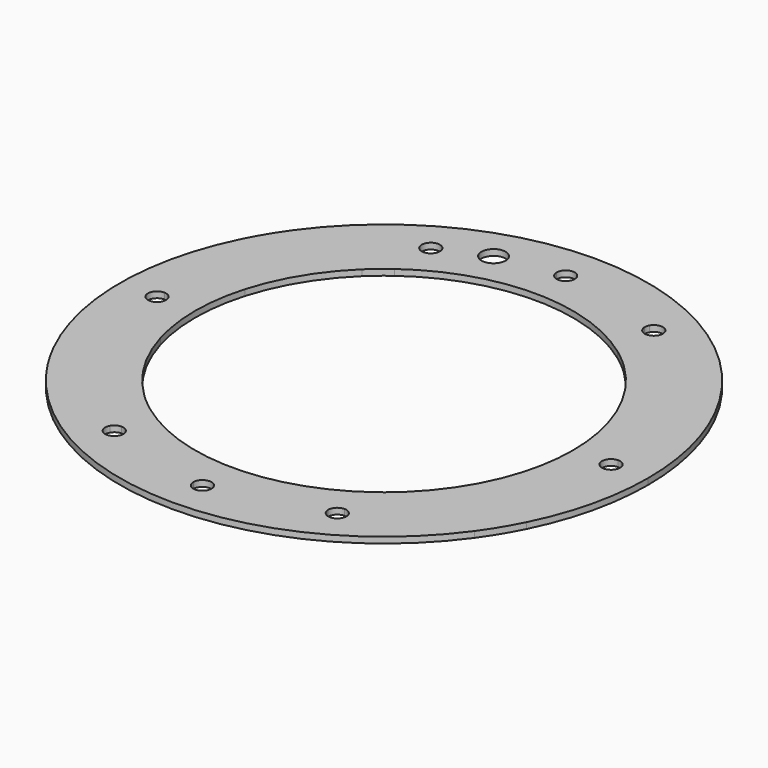
from build123d import *

# Parameters (mm, degrees)
F0_W     = 2.1041625413
F0_H     = 6.15
F1_DEPTH = 2


# Not quite as in the source:
# - a feature names something its author has since deleted; it is built from what else it names


with BuildPart() as f1:
    # F0 (on Top) → F1 (new body)
    with BuildSketch(Plane.XY):
        with Locations((59.2149618303, 40.7632449339)):
            Rectangle(F0_W, F0_H)
        with BuildLine():
            Line((58.1628805597, 43.8382449339), (60.2670431009, 43.8382449339))
            Line((60.2670431009, 43.8382449339), (60.2670431009, 37.6882449339))
            Line((60.2670431009, 37.6882449339), (62.3712056422, 37.6882449339))
            Line((62.3712056422, 37.6882449339), (62.3712056422, 41.1268579364))
            ThreePointArc((62.3712056422, 41.1268579364), (60.3323424952, 43.9759631228), (58.1628805597, 46.7269262644))
            Line((58.1628805597, 46.7269262644), (58.1628805597, 43.8382449339))
        make_face()
        with BuildLine():
            Line((58.1628805597, 37.6882449339), (58.1628805597, 43.8382449339))
            Line((58.1628805597, 43.8382449339), (53.7670431009, 43.8382449339))
            ThreePointArc((53.7670431009, 43.8382449339), (54.9789878574, 40.0585000032), (58.1628805597, 37.6882449339))
        make_face()
        with BuildLine():
            Line((53.7670431009, 43.8382449339), (58.1628805597, 43.8382449339))
            Line((58.1628805597, 43.8382449339), (58.1628805597, 46.7269262644))
            ThreePointArc((58.1628805597, 46.7269262644), (57.217639487, 47.8472580426), (56.25072261, 48.9489366399))
            ThreePointArc((56.25072261, 48.9489366399), (54.4208441995, 46.6793641507), (53.7670431009, 43.8382449339))
        make_face()
        with BuildLine():
            Line((62.3712056422, 37.6882449339), (60.2670431009, 37.6882449339))
            Line((60.2670431009, 37.6882449339), (60.2670431009, 37.3382449339))
            ThreePointArc((60.2670431009, 37.3382449339), (61.3335795513, 37.4263419402), (62.3712056422, 37.6882449339))
        make_face()
        with BuildLine():
            Line((60.2670431009, 37.3382449339), (60.2670431009, 37.6882449339))
            Line((60.2670431009, 37.6882449339), (58.1628805597, 37.6882449339))
            ThreePointArc((58.1628805597, 37.6882449339), (59.2005066506, 37.4263419402), (60.2670431009, 37.3382449339))
        make_face()
        with BuildLine():
            ThreePointArc((58.1628805597, 37.6882449339), (54.9789878574, 40.0585000032), (53.7670431009, 43.8382449339))
            Line((53.7670431009, 43.8382449339), (43.6404220332, 43.8382449339))
            ThreePointArc((43.6404220332, 43.8382449339), (53.7513993929, 31.1751222109), (60.2670431009, 16.3382449339))
            Line((60.2670431009, 16.3382449339), (60.2670431009, 37.3382449339))
            ThreePointArc((60.2670431009, 37.3382449339), (59.2005066506, 37.4263419402), (58.1628805597, 37.6882449339))
        make_face()
        with BuildLine():
            Line((43.6404220332, 43.8382449339), (53.7670431009, 43.8382449339))
            ThreePointArc((53.7670431009, 43.8382449339), (54.4208441995, 46.6793641507), (56.25072261, 48.9489366399))
            ThreePointArc((56.25072261, 48.9489366399), (48.4949826486, 56.4517818988), (39.7444489138, 62.7662374325))
            ThreePointArc((39.7444489138, 62.7662374325), (38.6484141737, 61.6859457367), (37.1609606052, 61.2912253535))
            Line((37.1609606052, 61.2912253535), (37.1609606052, 49.2871185703))
            ThreePointArc((37.1609606052, 49.2871185703), (40.4930580078, 46.6725184699), (43.6404220332, 43.8382449339))
        make_face()
        with BuildLine():
            ThreePointArc((56.25072261, 48.9489366399), (57.217639487, 47.8472580426), (58.1628805597, 46.7269262644))
            Line((58.1628805597, 46.7269262644), (58.1628805597, 49.9882449339))
            ThreePointArc((58.1628805597, 49.9882449339), (57.1629943627, 49.5491889391), (56.25072261, 48.9489366399))
        make_face()
        with BuildLine():
            Line((58.1628805597, 49.9882449339), (58.1628805597, 46.7269262644))
            ThreePointArc((58.1628805597, 46.7269262644), (60.3323424952, 43.9759631228), (62.3712056422, 41.1268579364))
            Line((62.3712056422, 41.1268579364), (62.3712056422, 49.9882449339))
            Line((62.3712056422, 49.9882449339), (58.1628805597, 49.9882449339))
        make_face()
        with BuildLine():
            ThreePointArc((62.3712056422, 37.6882449339), (61.3335795513, 37.4263419402), (60.2670431009, 37.3382449339))
            Line((60.2670431009, 37.3382449339), (60.2670431009, 16.3382449339))
            ThreePointArc((60.2670431009, 16.3382449339), (62.1388864548, 7.6770796987), (62.7670431009, -1.1617550661))
            ThreePointArc((62.7670431009, -1.1617550661), (62.1388864548, -10.000589831), (60.2670431009, -18.6617550661))
            Line((60.2670431009, -18.6617550661), (60.2670431009, -39.6617550661))
            ThreePointArc((60.2670431009, -39.6617550661), (61.3335795513, -39.7498520725), (62.3712056422, -40.0117550661))
            Line((62.3712056422, -40.0117550661), (64.5782497031, -40.0117550661))
            ThreePointArc((64.5782497031, -40.0117550661), (72.228412317, -22.7676601657), (75.3420410137, -4.1615022256))
            ThreePointArc((75.3420410137, -4.1615022256), (72.3809894341, -1.1617550661), (75.3420410137, 1.8379920933))
            ThreePointArc((75.3420410137, 1.8379920933), (72.228412317, 20.4441500334), (64.5782497031, 37.6882449339))
            Line((64.5782497031, 37.6882449339), (62.3712056422, 37.6882449339))
        make_face()
        with BuildLine():
            Line((62.3712056422, 41.1268579364), (62.3712056422, 37.6882449339))
            ThreePointArc((62.3712056422, 37.6882449339), (63.2414617158, 38.0587264501), (64.0487374012, 38.5515835849))
            ThreePointArc((64.0487374012, 38.5515835849), (63.2231408809, 39.8477992712), (62.3712056422, 41.1268579364))
        make_face()
        with BuildLine():
            ThreePointArc((64.0487374012, 38.5515835849), (63.2414617158, 38.0587264501), (62.3712056422, 37.6882449339))
            Line((62.3712056422, 37.6882449339), (64.5782497031, 37.6882449339))
            ThreePointArc((64.5782497031, 37.6882449339), (64.3149482486, 38.1208064697), (64.0487374012, 38.5515835849))
        make_face()
        with BuildLine():
            ThreePointArc((39.7444489138, 62.7662374325), (48.4949826486, 56.4517818988), (56.25072261, 48.9489366399))
            ThreePointArc((56.25072261, 48.9489366399), (57.1629943627, 49.5491889391), (58.1628805597, 49.9882449339))
            ThreePointArc((58.1628805597, 49.9882449339), (60.2670431009, 50.3382449339), (62.3712056422, 49.9882449339))
            Line((62.3712056422, 49.9882449339), (71.1075096636, 49.9882449339))
            ThreePointArc((71.1075096636, 49.9882449339), (0.2670431009, 86.2149821287), (-70.5734234617, 49.9882449339))
            Line((-70.5734234617, 49.9882449339), (-61.8371194403, 49.9882449339))
            ThreePointArc((-61.8371194403, 49.9882449339), (-59.7329568991, 50.3382449339), (-57.6287943578, 49.9882449339))
            ThreePointArc((-57.6287943578, 49.9882449339), (-56.6289081608, 49.5491889391), (-55.7166364081, 48.9489366399))
            ThreePointArc((-55.7166364081, 48.9489366399), (-47.9608964467, 56.4517818988), (-39.210362712, 62.7662374325))
            ThreePointArc((-39.210362712, 62.7662374325), (-38.0999813971, 66.9046437634), (-33.9845676129, 65.7118642328))
            ThreePointArc((-33.9845676129, 65.7118642328), (-29.5146570092, 67.8187069008), (-24.9159238599, 69.6271704072))
            ThreePointArc((-24.9159238599, 69.6271704072), (-22.2511598208, 74.7016983457), (-17.2493627904, 71.9028007682))
            ThreePointArc((-17.2493627904, 71.9028007682), (-10.040168129, 73.2628053376), (-2.7327040585, 73.9132428466))
            ThreePointArc((-2.7327040585, 73.9132428466), (0.2475684804, 76.9521280563), (3.2670431009, 73.9521912671))
            ThreePointArc((3.2670431009, 73.9521912671), (3.2669798901, 73.9327166465), (3.2667902604, 73.9132428466))
            ThreePointArc((3.2667902604, 73.9132428466), (19.3387910188, 71.5123271502), (34.5186538148, 65.7118642328))
            ThreePointArc((34.5186538148, 65.7118642328), (37.8934493863, 67.2004280253), (40.1609606052, 64.2912253535))
            ThreePointArc((40.1609606052, 64.2912253535), (40.0549599941, 63.5008029746), (39.7444489138, 62.7662374325))
        make_face()
        with BuildLine():
            ThreePointArc((62.3712056422, 49.9882449339), (60.2670431009, 50.3382449339), (58.1628805597, 49.9882449339))
            Line((58.1628805597, 49.9882449339), (62.3712056422, 49.9882449339))
        make_face()
        with BuildLine():
            Line((62.3712056422, 49.9882449339), (62.3712056422, 41.1268579364))
            ThreePointArc((62.3712056422, 41.1268579364), (63.2231408809, 39.8477992712), (64.0487374012, 38.5515835849))
            ThreePointArc((64.0487374012, 38.5515835849), (66.0476578153, 40.8659573428), (66.7670431009, 43.8382449339))
            ThreePointArc((66.7670431009, 43.8382449339), (65.5550983445, 47.6179898645), (62.3712056422, 49.9882449339))
        make_face()
        with BuildLine():
            ThreePointArc((66.7670431009, 43.8382449339), (66.0476578153, 40.8659573428), (64.0487374012, 38.5515835849))
            ThreePointArc((64.0487374012, 38.5515835849), (64.3149482486, 38.1208064697), (64.5782497031, 37.6882449339))
            Line((64.5782497031, 37.6882449339), (78.5317969996, 37.6882449339))
            ThreePointArc((78.5317969996, 37.6882449339), (75.0728864035, 43.9910965671), (71.1075096636, 49.9882449339))
            Line((71.1075096636, 49.9882449339), (62.3712056422, 49.9882449339))
            ThreePointArc((62.3712056422, 49.9882449339), (65.5550983445, 47.6179898645), (66.7670431009, 43.8382449339))
        make_face()
        with BuildLine():
            Line((78.5317969996, 37.6882449339), (64.5782497031, 37.6882449339))
            ThreePointArc((64.5782497031, 37.6882449339), (72.228412317, 20.4441500334), (75.3420410137, 1.8379920933))
            ThreePointArc((75.3420410137, 1.8379920933), (77.4884944447, 0.9732912169), (78.3809894341, -1.1617550661))
            ThreePointArc((78.3809894341, -1.1617550661), (77.4884944447, -3.2968013492), (75.3420410137, -4.1615022256))
            ThreePointArc((75.3420410137, -4.1615022256), (72.228412317, -22.7676601657), (64.5782497031, -40.0117550661))
            Line((64.5782497031, -40.0117550661), (78.5317969996, -40.0117550661))
            ThreePointArc((78.5317969996, -40.0117550661), (85.3352893384, -21.1138899118), (87.6437802958, -1.1617550661))
            ThreePointArc((87.6437802958, -1.1617550661), (85.3352893384, 18.7903797795), (78.5317969996, 37.6882449339))
        make_face()
        with BuildLine():
            ThreePointArc((-36.6268744033, 49.2871185703), (0.2670431009, 61.3382449339), (37.1609606052, 49.2871185703))
            Line((37.1609606052, 49.2871185703), (37.1609606052, 61.2912253535))
            ThreePointArc((37.1609606052, 61.2912253535), (35.0396402617, 62.1699050099), (34.1609606052, 64.2912253535))
            Line((34.1609606052, 64.2912253535), (-33.6268744033, 64.2912253535))
            ThreePointArc((-33.6268744033, 64.2912253535), (-34.5055540598, 62.1699050099), (-36.6268744033, 61.2912253535))
            Line((-36.6268744033, 61.2912253535), (-36.6268744033, 49.2871185703))
        make_face()
        with BuildLine():
            Line((60.2670431009, -39.6617550661), (60.2670431009, -18.6617550661))
            ThreePointArc((60.2670431009, -18.6617550661), (53.7513993929, -33.4986323432), (43.6404220332, -46.1617550661))
            Line((43.6404220332, -46.1617550661), (53.7670431009, -46.1617550661))
            ThreePointArc((53.7670431009, -46.1617550661), (54.9789878574, -42.3820101355), (58.1628805597, -40.0117550661))
            ThreePointArc((58.1628805597, -40.0117550661), (59.2005066506, -39.7498520725), (60.2670431009, -39.6617550661))
        make_face()
        with BuildLine():
            ThreePointArc((-43.1063358313, 43.8382449339), (-39.9589718059, 46.6725184699), (-36.6268744033, 49.2871185703))
            Line((-36.6268744033, 49.2871185703), (-36.6268744033, 61.2912253535))
            ThreePointArc((-36.6268744033, 61.2912253535), (-38.1143279719, 61.6859457367), (-39.210362712, 62.7662374325))
            ThreePointArc((-39.210362712, 62.7662374325), (-47.9608964467, 56.4517818988), (-55.7166364081, 48.9489366399))
            ThreePointArc((-55.7166364081, 48.9489366399), (-53.8867579976, 46.6793641507), (-53.2329568991, 43.8382449339))
            Line((-53.2329568991, 43.8382449339), (-43.1063358313, 43.8382449339))
        make_face()
        with BuildLine():
            ThreePointArc((62.3712056422, -40.0117550661), (61.3335795513, -39.7498520725), (60.2670431009, -39.6617550661))
            Line((60.2670431009, -39.6617550661), (60.2670431009, -40.0117550661))
            Line((60.2670431009, -40.0117550661), (62.3712056422, -40.0117550661))
        make_face()
        with BuildLine():
            Line((60.2670431009, -40.0117550661), (60.2670431009, -39.6617550661))
            ThreePointArc((60.2670431009, -39.6617550661), (59.2005066506, -39.7498520725), (58.1628805597, -40.0117550661))
            Line((58.1628805597, -40.0117550661), (60.2670431009, -40.0117550661))
        make_face()
        with BuildLine():
            Line((53.7670431009, -46.1617550661), (43.6404220332, -46.1617550661))
            ThreePointArc((43.6404220332, -46.1617550661), (40.4930580078, -48.9960286021), (37.1609606052, -51.6106287026))
            Line((37.1609606052, -51.6106287026), (37.1609606052, -63.6147354858))
            ThreePointArc((37.1609606052, -63.6147354858), (38.6484141737, -64.009455869), (39.7444489138, -65.0897475648))
            ThreePointArc((39.7444489138, -65.0897475648), (48.4949826486, -58.7752920311), (56.25072261, -51.2724467721))
            ThreePointArc((56.25072261, -51.2724467721), (54.4208441995, -49.002874283), (53.7670431009, -46.1617550661))
        make_face()
        with BuildLine():
            ThreePointArc((-59.7329568991, 16.3382449339), (-53.217313191, 31.1751222109), (-43.1063358313, 43.8382449339))
            Line((-43.1063358313, 43.8382449339), (-53.2329568991, 43.8382449339))
            ThreePointArc((-53.2329568991, 43.8382449339), (-54.4449016555, 40.0585000032), (-57.6287943578, 37.6882449339))
            ThreePointArc((-57.6287943578, 37.6882449339), (-58.6664204487, 37.4263419402), (-59.7329568991, 37.3382449339))
            Line((-59.7329568991, 37.3382449339), (-59.7329568991, 16.3382449339))
        make_face()
        with BuildLine():
            Line((37.1609606052, -63.6147354858), (37.1609606052, -51.6106287026))
            ThreePointArc((37.1609606052, -51.6106287026), (0.2670431009, -63.6617550661), (-36.6268744033, -51.6106287026))
            Line((-36.6268744033, -51.6106287026), (-36.6268744033, -63.6147354858))
            ThreePointArc((-36.6268744033, -63.6147354858), (-34.5055540598, -64.4934151422), (-33.6268744033, -66.6147354858))
            Line((-33.6268744033, -66.6147354858), (34.1609606052, -66.6147354858))
            ThreePointArc((34.1609606052, -66.6147354858), (35.0396402617, -64.4934151422), (37.1609606052, -63.6147354858))
        make_face()
        with BuildLine():
            Line((-33.6268744033, 64.2912253535), (34.1609606052, 64.2912253535))
            ThreePointArc((34.1609606052, 64.2912253535), (34.2517579334, 65.0237141345), (34.5186538148, 65.7118642328))
            ThreePointArc((34.5186538148, 65.7118642328), (19.3387910188, 71.5123271502), (3.2667902604, 73.9132428466))
            ThreePointArc((3.2667902604, 73.9132428466), (0.2670431009, 70.9521912671), (-2.7327040585, 73.9132428466))
            ThreePointArc((-2.7327040585, 73.9132428466), (-10.040168129, 73.2628053376), (-17.2493627904, 71.9028007682))
            ThreePointArc((-17.2493627904, 71.9028007682), (-17.1471933384, 71.3894027327), (-17.1129413209, 70.8670590345))
            ThreePointArc((-17.1129413209, 70.8670590345), (-20.4852193108, 66.9166204414), (-24.9159238599, 69.6271704072))
            ThreePointArc((-24.9159238599, 69.6271704072), (-29.5146570092, 67.8187069008), (-33.9845676129, 65.7118642328))
            ThreePointArc((-33.9845676129, 65.7118642328), (-33.7176717315, 65.0237141345), (-33.6268744033, 64.2912253535))
        make_face()
        with BuildLine():
            Line((-61.8371194403, 49.9882449339), (-70.5734234617, 49.9882449339))
            ThreePointArc((-70.5734234617, 49.9882449339), (-74.5388002016, 43.9910965671), (-77.9977107977, 37.6882449339))
            Line((-77.9977107977, 37.6882449339), (-64.0441635012, 37.6882449339))
            ThreePointArc((-64.0441635012, 37.6882449339), (-63.7808620468, 38.1208064697), (-63.5146511994, 38.5515835849))
            ThreePointArc((-63.5146511994, 38.5515835849), (-66.1641413462, 44.7815723464), (-61.8371194403, 49.9882449339))
        make_face()
        with BuildLine():
            Line((62.3712056422, -40.0117550661), (60.2670431009, -40.0117550661))
            Line((60.2670431009, -40.0117550661), (60.2670431009, -46.1617550661))
            Line((60.2670431009, -46.1617550661), (58.1628805597, -46.1617550661))
            Line((58.1628805597, -46.1617550661), (58.1628805597, -49.0504363967))
            ThreePointArc((58.1628805597, -49.0504363967), (60.3323424952, -46.2994732551), (62.3712056422, -43.4503680686))
            Line((62.3712056422, -43.4503680686), (62.3712056422, -40.0117550661))
        make_face()
        with Locations((59.2149618303, -43.0867550661)):
            Rectangle(F0_W, F0_H)
        with BuildLine():
            Line((64.5782497031, -40.0117550661), (62.3712056422, -40.0117550661))
            ThreePointArc((62.3712056422, -40.0117550661), (63.2414617158, -40.3822365824), (64.0487374012, -40.8750937171))
            ThreePointArc((64.0487374012, -40.8750937171), (64.3149482486, -40.444316602), (64.5782497031, -40.0117550661))
        make_face()
        with BuildLine():
            ThreePointArc((64.0487374012, -40.8750937171), (63.2414617158, -40.3822365824), (62.3712056422, -40.0117550661))
            Line((62.3712056422, -40.0117550661), (62.3712056422, -43.4503680686))
            ThreePointArc((62.3712056422, -43.4503680686), (63.2231408809, -42.1713094035), (64.0487374012, -40.8750937171))
        make_face()
        with BuildLine():
            Line((58.1628805597, -46.1617550661), (58.1628805597, -40.0117550661))
            ThreePointArc((58.1628805597, -40.0117550661), (54.9789878574, -42.3820101355), (53.7670431009, -46.1617550661))
            Line((53.7670431009, -46.1617550661), (58.1628805597, -46.1617550661))
        make_face()
        with BuildLine():
            Line((58.1628805597, -46.1617550661), (53.7670431009, -46.1617550661))
            ThreePointArc((53.7670431009, -46.1617550661), (54.4208441995, -49.002874283), (56.25072261, -51.2724467721))
            ThreePointArc((56.25072261, -51.2724467721), (57.217639487, -50.1707681749), (58.1628805597, -49.0504363967))
            Line((58.1628805597, -49.0504363967), (58.1628805597, -46.1617550661))
        make_face()
        with BuildLine():
            ThreePointArc((71.1075096636, -52.3117550661), (75.0728864035, -46.3146066994), (78.5317969996, -40.0117550661))
            Line((78.5317969996, -40.0117550661), (64.5782497031, -40.0117550661))
            ThreePointArc((64.5782497031, -40.0117550661), (64.3149482486, -40.444316602), (64.0487374012, -40.8750937171))
            ThreePointArc((64.0487374012, -40.8750937171), (66.0476578153, -43.1894674751), (66.7670431009, -46.1617550661))
            ThreePointArc((66.7670431009, -46.1617550661), (65.5550983445, -49.9414999968), (62.3712056422, -52.3117550661))
            Line((62.3712056422, -52.3117550661), (71.1075096636, -52.3117550661))
        make_face()
        with BuildLine():
            ThreePointArc((-57.6287943578, 37.6882449339), (-54.4449016555, 40.0585000032), (-53.2329568991, 43.8382449339))
            Line((-53.2329568991, 43.8382449339), (-57.6287943578, 43.8382449339))
            Line((-57.6287943578, 43.8382449339), (-57.6287943578, 37.6882449339))
        make_face()
        with BuildLine():
            Line((-57.6287943578, 43.8382449339), (-53.2329568991, 43.8382449339))
            ThreePointArc((-53.2329568991, 43.8382449339), (-53.8867579976, 46.6793641507), (-55.7166364081, 48.9489366399))
            ThreePointArc((-55.7166364081, 48.9489366399), (-56.6835532851, 47.8472580426), (-57.6287943578, 46.7269262644))
            Line((-57.6287943578, 46.7269262644), (-57.6287943578, 43.8382449339))
        make_face()
        with BuildLine():
            ThreePointArc((-59.7329568991, -18.6617550661), (-62.2329568991, -1.1617550661), (-59.7329568991, 16.3382449339))
            Line((-59.7329568991, 16.3382449339), (-59.7329568991, 37.3382449339))
            ThreePointArc((-59.7329568991, 37.3382449339), (-60.7994933494, 37.4263419402), (-61.8371194403, 37.6882449339))
            Line((-61.8371194403, 37.6882449339), (-64.0441635012, 37.6882449339))
            ThreePointArc((-64.0441635012, 37.6882449339), (-71.6943261151, 20.4441500334), (-74.8079548118, 1.8379920933))
            ThreePointArc((-74.8079548118, 1.8379920933), (-72.7118569492, 0.9457499444), (-71.8469032323, -1.1617550661))
            ThreePointArc((-71.8469032323, -1.1617550661), (-72.7118569492, -3.2692600767), (-74.8079548118, -4.1615022256))
            ThreePointArc((-74.8079548118, -4.1615022256), (-71.6943261151, -22.7676601657), (-64.0441635012, -40.0117550661))
            Line((-64.0441635012, -40.0117550661), (-61.8371194403, -40.0117550661))
            ThreePointArc((-61.8371194403, -40.0117550661), (-60.7994933494, -39.7498520725), (-59.7329568991, -39.6617550661))
            Line((-59.7329568991, -39.6617550661), (-59.7329568991, -18.6617550661))
        make_face()
        with BuildLine():
            ThreePointArc((-36.6268744033, -51.6106287026), (-39.9589718059, -48.9960286021), (-43.1063358313, -46.1617550661))
            Line((-43.1063358313, -46.1617550661), (-53.2329568991, -46.1617550661))
            ThreePointArc((-53.2329568991, -46.1617550661), (-53.8867579976, -49.002874283), (-55.7166364081, -51.2724467721))
            ThreePointArc((-55.7166364081, -51.2724467721), (-47.9608964467, -58.7752920311), (-39.210362712, -65.0897475648))
            ThreePointArc((-39.210362712, -65.0897475648), (-38.1143279719, -64.009455869), (-36.6268744033, -63.6147354858))
            Line((-36.6268744033, -63.6147354858), (-36.6268744033, -51.6106287026))
        make_face()
        with BuildLine():
            Line((-53.2329568991, -46.1617550661), (-43.1063358313, -46.1617550661))
            ThreePointArc((-43.1063358313, -46.1617550661), (-53.217313191, -33.4986323432), (-59.7329568991, -18.6617550661))
            Line((-59.7329568991, -18.6617550661), (-59.7329568991, -39.6617550661))
            ThreePointArc((-59.7329568991, -39.6617550661), (-58.6664204487, -39.7498520725), (-57.6287943578, -40.0117550661))
            ThreePointArc((-57.6287943578, -40.0117550661), (-54.4449016555, -42.3820101355), (-53.2329568991, -46.1617550661))
        make_face()
        with BuildLine():
            Line((-64.0441635012, 37.6882449339), (-77.9977107977, 37.6882449339))
            ThreePointArc((-77.9977107977, 37.6882449339), (-87.1096939106, -1.1674142446), (-77.9926777014, -40.0218927752))
            Line((-77.9926777014, -40.0218927752), (-77.9926777014, -40.0117550661))
            Line((-77.9926777014, -40.0117550661), (-64.0441635012, -40.0117550661))
            ThreePointArc((-64.0441635012, -40.0117550661), (-71.6943261151, -22.7676601657), (-74.8079548118, -4.1615022256))
            ThreePointArc((-74.8079548118, -4.1615022256), (-77.8469032323, -1.1617550661), (-74.8079548118, 1.8379920933))
            ThreePointArc((-74.8079548118, 1.8379920933), (-71.6943261151, 20.4441500334), (-64.0441635012, 37.6882449339))
        make_face()
        with BuildLine():
            Line((-61.8371194403, 41.1268579364), (-61.8371194403, 49.9882449339))
            ThreePointArc((-61.8371194403, 49.9882449339), (-66.1641413462, 44.7815723464), (-63.5146511994, 38.5515835849))
            ThreePointArc((-63.5146511994, 38.5515835849), (-62.689054679, 39.8477992712), (-61.8371194403, 41.1268579364))
        make_face()
        with BuildLine():
            ThreePointArc((-57.6287943578, 49.9882449339), (-59.7329568991, 50.3382449339), (-61.8371194403, 49.9882449339))
            Line((-61.8371194403, 49.9882449339), (-57.6287943578, 49.9882449339))
        make_face()
        with BuildLine():
            Line((-57.6287943578, 49.9882449339), (-61.8371194403, 49.9882449339))
            Line((-61.8371194403, 49.9882449339), (-61.8371194403, 41.1268579364))
            ThreePointArc((-61.8371194403, 41.1268579364), (-59.7982562933, 43.9759631228), (-57.6287943578, 46.7269262644))
            Line((-57.6287943578, 46.7269262644), (-57.6287943578, 49.9882449339))
        make_face()
        with BuildLine():
            ThreePointArc((66.7670431009, -46.1617550661), (66.0476578153, -43.1894674751), (64.0487374012, -40.8750937171))
            ThreePointArc((64.0487374012, -40.8750937171), (63.2231408809, -42.1713094035), (62.3712056422, -43.4503680686))
            Line((62.3712056422, -43.4503680686), (62.3712056422, -52.3117550661))
            ThreePointArc((62.3712056422, -52.3117550661), (65.5550983445, -49.9414999968), (66.7670431009, -46.1617550661))
        make_face()
        with BuildLine():
            Line((62.3712056422, -52.3117550661), (62.3712056422, -43.4503680686))
            ThreePointArc((62.3712056422, -43.4503680686), (60.3323424952, -46.2994732551), (58.1628805597, -49.0504363967))
            Line((58.1628805597, -49.0504363967), (58.1628805597, -52.3117550661))
            Line((58.1628805597, -52.3117550661), (62.3712056422, -52.3117550661))
        make_face()
        with BuildLine():
            ThreePointArc((58.1628805597, -49.0504363967), (57.217639487, -50.1707681749), (56.25072261, -51.2724467721))
            ThreePointArc((56.25072261, -51.2724467721), (57.1629943627, -51.8726990713), (58.1628805597, -52.3117550661))
            Line((58.1628805597, -52.3117550661), (58.1628805597, -49.0504363967))
        make_face()
        with BuildLine():
            ThreePointArc((58.1628805597, -52.3117550661), (57.1629943627, -51.8726990713), (56.25072261, -51.2724467721))
            ThreePointArc((56.25072261, -51.2724467721), (48.4949826486, -58.7752920311), (39.7444489138, -65.0897475648))
            ThreePointArc((39.7444489138, -65.0897475648), (40.0549599941, -65.8243131069), (40.1609606052, -66.6147354858))
            ThreePointArc((40.1609606052, -66.6147354858), (37.8934493863, -69.5239381576), (34.5186538148, -68.035374365))
            ThreePointArc((34.5186538148, -68.035374365), (19.3387910188, -73.8358372824), (3.2667902604, -76.2367529789))
            ThreePointArc((3.2667902604, -76.2367529789), (3.2669798901, -76.2562267788), (3.2670431009, -76.2757013993))
            ThreePointArc((3.2670431009, -76.2757013993), (0.2475684804, -79.2756381885), (-2.7327040585, -76.2367529789))
            ThreePointArc((-2.7327040585, -76.2367529789), (-18.8047048169, -73.8358372824), (-33.9845676129, -68.035374365))
            ThreePointArc((-33.9845676129, -68.035374365), (-38.0999813971, -69.2281538956), (-39.210362712, -65.0897475648))
            ThreePointArc((-39.210362712, -65.0897475648), (-47.9608964467, -58.7752920311), (-55.7166364081, -51.2724467721))
            ThreePointArc((-55.7166364081, -51.2724467721), (-56.6289081608, -51.8726990713), (-57.6287943578, -52.3117550661))
            ThreePointArc((-57.6287943578, -52.3117550661), (-59.7329568991, -52.6617550661), (-61.8371194403, -52.3117550661))
            Line((-61.8371194403, -52.3117550661), (-70.5734234617, -52.3117550661))
            ThreePointArc((-70.5734234617, -52.3117550661), (0.2670431009, -88.538492261), (71.1075096636, -52.3117550661))
            Line((71.1075096636, -52.3117550661), (62.3712056422, -52.3117550661))
            ThreePointArc((62.3712056422, -52.3117550661), (60.2670431009, -52.6617550661), (58.1628805597, -52.3117550661))
        make_face()
        with Locations((-58.6808756284, 40.7632449339)):
            Rectangle(F0_W, F0_H)
        with BuildLine():
            Line((-59.7329568991, 43.8382449339), (-57.6287943578, 43.8382449339))
            Line((-57.6287943578, 43.8382449339), (-57.6287943578, 46.7269262644))
            ThreePointArc((-57.6287943578, 46.7269262644), (-59.7982562933, 43.9759631228), (-61.8371194403, 41.1268579364))
            Line((-61.8371194403, 41.1268579364), (-61.8371194403, 37.6882449339))
            Line((-61.8371194403, 37.6882449339), (-59.7329568991, 37.6882449339))
            Line((-59.7329568991, 37.6882449339), (-59.7329568991, 43.8382449339))
        make_face()
        with BuildLine():
            ThreePointArc((-59.7329568991, 37.3382449339), (-58.6664204487, 37.4263419402), (-57.6287943578, 37.6882449339))
            Line((-57.6287943578, 37.6882449339), (-59.7329568991, 37.6882449339))
            Line((-59.7329568991, 37.6882449339), (-59.7329568991, 37.3382449339))
        make_face()
        with BuildLine():
            ThreePointArc((-57.6287943578, 46.7269262644), (-56.6835532851, 47.8472580426), (-55.7166364081, 48.9489366399))
            ThreePointArc((-55.7166364081, 48.9489366399), (-56.6289081608, 49.5491889391), (-57.6287943578, 49.9882449339))
            Line((-57.6287943578, 49.9882449339), (-57.6287943578, 46.7269262644))
        make_face()
        with BuildLine():
            ThreePointArc((-61.8371194403, 37.6882449339), (-60.7994933494, 37.4263419402), (-59.7329568991, 37.3382449339))
            Line((-59.7329568991, 37.3382449339), (-59.7329568991, 37.6882449339))
            Line((-59.7329568991, 37.6882449339), (-61.8371194403, 37.6882449339))
        make_face()
        with BuildLine():
            ThreePointArc((-55.7166364081, -51.2724467721), (-53.8867579976, -49.002874283), (-53.2329568991, -46.1617550661))
            Line((-53.2329568991, -46.1617550661), (-57.6287943578, -46.1617550661))
            Line((-57.6287943578, -46.1617550661), (-57.6287943578, -49.0504363967))
            ThreePointArc((-57.6287943578, -49.0504363967), (-56.6835532851, -50.1707681749), (-55.7166364081, -51.2724467721))
        make_face()
        with BuildLine():
            Line((-57.6287943578, -46.1617550661), (-53.2329568991, -46.1617550661))
            ThreePointArc((-53.2329568991, -46.1617550661), (-54.4449016555, -42.3820101355), (-57.6287943578, -40.0117550661))
            Line((-57.6287943578, -40.0117550661), (-57.6287943578, -46.1617550661))
        make_face()
        with BuildLine():
            ThreePointArc((34.5186538148, -68.035374365), (34.2517579334, -67.3472242668), (34.1609606052, -66.6147354858))
            Line((34.1609606052, -66.6147354858), (-33.6268744033, -66.6147354858))
            ThreePointArc((-33.6268744033, -66.6147354858), (-33.7176717315, -67.3472242668), (-33.9845676129, -68.035374365))
            ThreePointArc((-33.9845676129, -68.035374365), (-18.8047048169, -73.8358372824), (-2.7327040585, -76.2367529789))
            ThreePointArc((-2.7327040585, -76.2367529789), (0.2670431009, -73.2757013993), (3.2667902604, -76.2367529789))
            ThreePointArc((3.2667902604, -76.2367529789), (19.3387910188, -73.8358372824), (34.5186538148, -68.035374365))
        make_face()
        with BuildLine():
            Line((-77.9926777014, -40.0117550661), (-77.9926777014, -40.0218927752))
            ThreePointArc((-77.9926777014, -40.0218927752), (-74.5358756045, -46.3194515969), (-70.5734234617, -52.3117550661))
            Line((-70.5734234617, -52.3117550661), (-61.8371194403, -52.3117550661))
            ThreePointArc((-61.8371194403, -52.3117550661), (-66.1641413462, -47.1050824787), (-63.5146511994, -40.8750937171))
            ThreePointArc((-63.5146511994, -40.8750937171), (-63.7808620468, -40.444316602), (-64.0441635012, -40.0117550661))
            Line((-64.0441635012, -40.0117550661), (-77.9926777014, -40.0117550661))
        make_face()
        with BuildLine():
            ThreePointArc((-63.5146511994, 38.5515835849), (-63.7808620468, 38.1208064697), (-64.0441635012, 37.6882449339))
            Line((-64.0441635012, 37.6882449339), (-61.8371194403, 37.6882449339))
            ThreePointArc((-61.8371194403, 37.6882449339), (-62.7073755139, 38.0587264501), (-63.5146511994, 38.5515835849))
        make_face()
        with BuildLine():
            ThreePointArc((-61.8371194403, 41.1268579364), (-62.689054679, 39.8477992712), (-63.5146511994, 38.5515835849))
            ThreePointArc((-63.5146511994, 38.5515835849), (-62.7073755139, 38.0587264501), (-61.8371194403, 37.6882449339))
            Line((-61.8371194403, 37.6882449339), (-61.8371194403, 41.1268579364))
        make_face()
        with BuildLine():
            ThreePointArc((58.1628805597, -52.3117550661), (60.2670431009, -52.6617550661), (62.3712056422, -52.3117550661))
            Line((62.3712056422, -52.3117550661), (58.1628805597, -52.3117550661))
        make_face()
        with BuildLine():
            ThreePointArc((-57.6287943578, -40.0117550661), (-58.6664204487, -39.7498520725), (-59.7329568991, -39.6617550661))
            Line((-59.7329568991, -39.6617550661), (-59.7329568991, -40.0117550661))
            Line((-59.7329568991, -40.0117550661), (-57.6287943578, -40.0117550661))
        make_face()
        with BuildLine():
            Line((-59.7329568991, -40.0117550661), (-59.7329568991, -39.6617550661))
            ThreePointArc((-59.7329568991, -39.6617550661), (-60.7994933494, -39.7498520725), (-61.8371194403, -40.0117550661))
            Line((-61.8371194403, -40.0117550661), (-59.7329568991, -40.0117550661))
        make_face()
        with BuildLine():
            Line((-57.6287943578, -49.0504363967), (-57.6287943578, -46.1617550661))
            Line((-57.6287943578, -46.1617550661), (-59.7329568991, -46.1617550661))
            Line((-59.7329568991, -46.1617550661), (-59.7329568991, -40.0117550661))
            Line((-59.7329568991, -40.0117550661), (-61.8371194403, -40.0117550661))
            Line((-61.8371194403, -40.0117550661), (-61.8371194403, -43.4503680686))
            ThreePointArc((-61.8371194403, -43.4503680686), (-59.7982562933, -46.2994732551), (-57.6287943578, -49.0504363967))
        make_face()
        with Locations((-58.6808756284, -43.0867550661)):
            Rectangle(F0_W, F0_H)
        with BuildLine():
            ThreePointArc((-57.6287943578, -52.3117550661), (-56.6289081608, -51.8726990713), (-55.7166364081, -51.2724467721))
            ThreePointArc((-55.7166364081, -51.2724467721), (-56.6835532851, -50.1707681749), (-57.6287943578, -49.0504363967))
            Line((-57.6287943578, -49.0504363967), (-57.6287943578, -52.3117550661))
        make_face()
        with BuildLine():
            Line((-57.6287943578, -52.3117550661), (-61.8371194403, -52.3117550661))
            ThreePointArc((-61.8371194403, -52.3117550661), (-59.7329568991, -52.6617550661), (-57.6287943578, -52.3117550661))
        make_face()
        with BuildLine():
            Line((-61.8371194403, -43.4503680686), (-61.8371194403, -52.3117550661))
            Line((-61.8371194403, -52.3117550661), (-57.6287943578, -52.3117550661))
            Line((-57.6287943578, -52.3117550661), (-57.6287943578, -49.0504363967))
            ThreePointArc((-57.6287943578, -49.0504363967), (-59.7982562933, -46.2994732551), (-61.8371194403, -43.4503680686))
        make_face()
        with BuildLine():
            ThreePointArc((-63.5146511994, -40.8750937171), (-66.1641413462, -47.1050824787), (-61.8371194403, -52.3117550661))
            Line((-61.8371194403, -52.3117550661), (-61.8371194403, -43.4503680686))
            ThreePointArc((-61.8371194403, -43.4503680686), (-62.689054679, -42.1713094035), (-63.5146511994, -40.8750937171))
        make_face()
        with BuildLine():
            Line((-61.8371194403, -43.4503680686), (-61.8371194403, -40.0117550661))
            ThreePointArc((-61.8371194403, -40.0117550661), (-62.7073755139, -40.3822365824), (-63.5146511994, -40.8750937171))
            ThreePointArc((-63.5146511994, -40.8750937171), (-62.689054679, -42.1713094035), (-61.8371194403, -43.4503680686))
        make_face()
        with BuildLine():
            ThreePointArc((-63.5146511994, -40.8750937171), (-62.7073755139, -40.3822365824), (-61.8371194403, -40.0117550661))
            Line((-61.8371194403, -40.0117550661), (-64.0441635012, -40.0117550661))
            ThreePointArc((-64.0441635012, -40.0117550661), (-63.7808620468, -40.444316602), (-63.5146511994, -40.8750937171))
        make_face()
    extrude(amount=F1_DEPTH)


solid = f1.part
